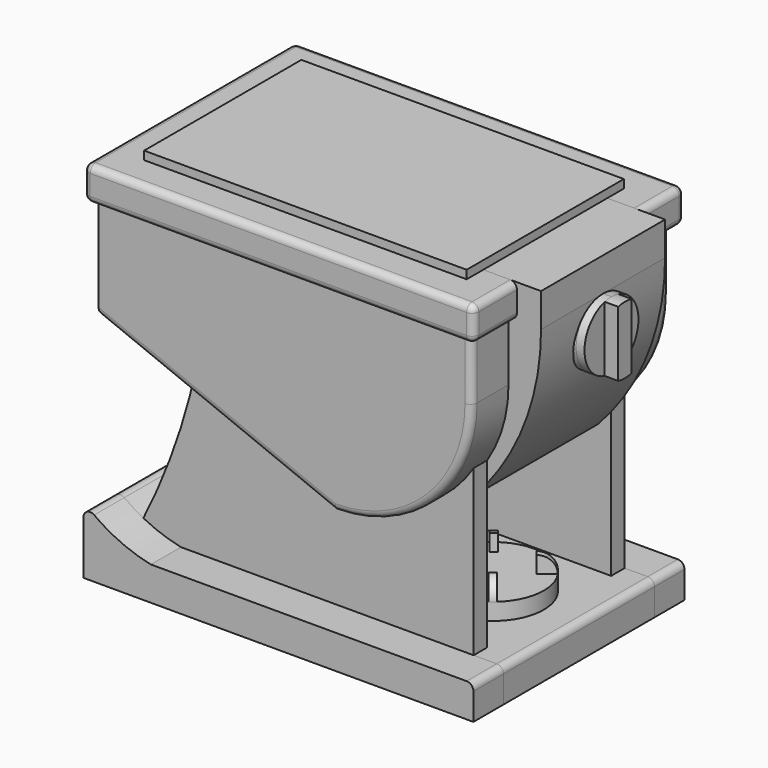
from build123d import *

# Parameters (mm, degrees)
F1_DEPTH       = 25.4
F2_W           = 140.589
F2_H           = 76.2
F3_DEPTH       = 93.091
F3_DEPTH_BACK  = 93.091
F5_DEPTH       = 99.441
F5_DEPTH_BACK  = 99.441
F4_W           = 124.46
F4_H           = 224.282
F6_DEPTH       = 71.12
F6_DEPTH_BACK  = 71.12
F7_R           = 103.37799
F9_R           = 5.08
F10_T1_DEPTH   = 203.3103950373
F10_T3_DEPTH   = 217.1807652608
F10_T5_DEPTH   = 44.70401
F10_T7_DEPTH   = 12.70001
F10_T10_ANGLE  = 90
F10_T12_ANGLE  = 90
F10_2_F1_R     = 5.08
F10_2_F2_R     = 5.08
F10_3_F1_R     = 5.08
F10_3_F2_R     = 5.08
F11_W          = 243.078
F11_H          = 148.082
F12_DEPTH      = 6.35
F13_DEPTH      = 101.6
F13_DEPTH_BACK = 25.4
F14_W          = 165.1
F14_H          = 25.4
F15_DEPTH      = 58.42
F15_DEPTH_BACK = 58.42
F17_DEPTH      = 6.35
F17_DEPTH_BACK = 25.4
F19_DEPTH      = 10.16
F21_DEPTH      = 12.7
F23_DEPTH      = 12.7
F24_T2_ANGLE   = 103.1383500352
F24_T4_ANGLE   = 103.1383500352
F24_T6_ANGLE   = 103.1383500352
F24_T8_ANGLE   = 103.1383500352


# Not quite as in the source:
# - a fillet or chamfer that OpenCascade refuses, or shapes differently, is made with other operations: its cross-section is extruded or revolved along the edge and cut away or added
# - a fillet or chamfer is up to 0.001 mm smaller than in the source, because OpenCascade refuses the exact size


with BuildPart() as f1:
    # F0 (on Top) → F1 (new body)
    with BuildSketch(Plane.XY):
        Polygon((146.939, 99.441), (0, 99.441), (-146.939, 99.441), (-146.939, 0), (-146.939, -99.441), (0, -99.441), (146.939, -99.441), (146.939, 0), align=None)
    extrude(amount=F1_DEPTH)

    # F2 (on Front) → F3 (join, two sides)
    with BuildSketch(Plane.XZ) as f3_sk:
        with Locations((-70.2945, -38.1)):
            Rectangle(F2_W, F2_H)
        Polygon((140.589, 0), (0, 0), (0, -76.2), (-140.589, -76.2), (37.211, -148.082), (140.589, -148.082), align=None)
    extrude(amount=F3_DEPTH)
    extrude(f3_sk.sketch, amount=-F3_DEPTH_BACK)

    # F7 (radius 103.378 in the source; OpenCascade refuses exactly that, so slightly less here)
    f7_edges = [f1.edges().sort_by_distance(p)[0] for p in [
        (140.589, 0, -148.082),
    ]]
    fillet(f7_edges, radius=F7_R)

    # F9
    f9_edges = [f1.edges().sort_by_distance(p)[0] for p in [
        (0, 99.441, 25.4),
        (-146.939, 0, 25.4),
        (0, -99.441, 25.4),
        (146.939, 0, 25.4),
        (0, -99.441, 0),
        (-146.939, 0, 0),
        (146.939, -99.441, 12.7),
        (146.939, 99.441, 12.7),
        (146.939, 0, 0),
        (-146.939, 99.441, 12.7),
        (-146.939, -99.441, 12.7),
        (0, 99.441, 0),
    ]]
    fillet(f9_edges, radius=F9_R)

    # F10: fillet of radius 5.08 on 7 edges, made by hand

    # F10_s2 → F10_t1 (cut)
    with BuildSketch(Plane.XZ.offset(-101.6551975186)):
        with BuildLine():
            ThreePointArc((-140.589, -72.7743209925), (-139.7208276576, -75.6145512267), (-137.4130520539, -77.4839903839))
            Line((-137.4130520539, -77.4839903839), (-140.589, -76.2))
            Line((-140.589, -76.2), (-140.589, -72.7743209925))
        make_face()
    extrude(amount=F10_T1_DEPTH, mode=Mode.SUBTRACT)

    # F10_s4 → F10_t3 (cut)
    with BuildSketch(Plane(origin=(-106.1338085529, 0, 42.9083826007), x_dir=(0, 1, 0), z_dir=(0.9271002739, 0, -0.3748133964))):
        with BuildLine():
            ThreePointArc((-93.091, -118.259681463), (-91.6031024484, -121.8517839115), (-88.011, -123.339681463))
            Line((-88.011, -123.339681463), (-93.091, -123.339681463))
            Line((-93.091, -123.339681463), (-93.091, -118.259681463))
        make_face()
        with BuildLine():
            ThreePointArc((93.091, -118.259681463), (91.6031024484, -121.8517839115), (88.011, -123.339681463))
            Line((88.011, -123.339681463), (93.091, -123.339681463))
            Line((93.091, -123.339681463), (93.091, -118.259681463))
        make_face()
    extrude(amount=F10_T3_DEPTH, mode=Mode.SUBTRACT)

    # F10_s6 → F10_t5 (cut)
    with BuildSketch(Plane.XY.offset(-44.70401)):
        with BuildLine():
            ThreePointArc((135.509, -93.091), (139.1011024484, -91.6031024484), (140.589, -88.011))
            Line((140.589, -88.011), (140.589, -93.091))
            Line((140.589, -93.091), (135.509, -93.091))
        make_face()
        with BuildLine():
            ThreePointArc((140.589, 88.011), (139.1011024484, 91.6031024484), (135.509, 93.091))
            Line((135.509, 93.091), (140.589, 93.091))
            Line((140.589, 93.091), (140.589, 88.011))
        make_face()
    extrude(amount=F10_T5_DEPTH, mode=Mode.SUBTRACT)

    # F10_s8 → F10_t7 (cut)
    with BuildSketch(Plane.YZ.offset(24.511)):
        with BuildLine():
            ThreePointArc((-93.091, -143.002), (-91.6031024484, -146.5941024484), (-88.011, -148.082))
            Line((-88.011, -148.082), (-93.091, -148.082))
            Line((-93.091, -148.082), (-93.091, -143.002))
        make_face()
        with BuildLine():
            ThreePointArc((93.091, -143.002), (91.6031024484, -146.5941024484), (88.011, -148.082))
            Line((88.011, -148.082), (93.091, -148.082))
            Line((93.091, -148.082), (93.091, -143.002))
        make_face()
    extrude(amount=F10_T7_DEPTH, mode=Mode.SUBTRACT)

    # F10_s9 → F10_t10 (revolve, cut)
    with BuildSketch(Plane.XY.offset(-44.70401)):
        with BuildLine():
            ThreePointArc((135.509, 93.091), (139.1011024484, 91.6031024484), (140.589, 88.011))
            Line((140.589, 88.011), (140.589, 93.091))
            Line((140.589, 93.091), (135.509, 93.091))
        make_face()
    revolve(axis=Axis((37.21101, 93.091, -44.70401), (0, 1, 0)), revolution_arc=F10_T10_ANGLE, mode=Mode.SUBTRACT)

    # F10_s11 → F10_t12 (revolve, cut)
    with BuildSketch(Plane.XY.offset(-44.70401)):
        with BuildLine():
            ThreePointArc((135.509, -93.091), (139.1011024484, -91.6031024484), (140.589, -88.011))
            Line((140.589, -88.011), (140.589, -93.091))
            Line((140.589, -93.091), (135.509, -93.091))
        make_face()
    revolve(axis=Axis((37.21101, -93.091, -44.70401), (0, 1, 0)), revolution_arc=F10_T12_ANGLE, mode=Mode.SUBTRACT)

    # F11 (on face) → F12 (join)
    with BuildSketch(Plane.XY.offset(25.4)):
        Rectangle(F11_W, F11_H)
    extrude(amount=F12_DEPTH)


with BuildPart() as f5:
    # F4 (on Front) → F5 (new body, two sides)
    with BuildSketch(Plane.XZ) as f5_sk:
        with BuildLine():
            Line((124.46, -224.282), (0, -224.282))
            Line((0, -224.282), (-96.139, -224.282))
            ThreePointArc((-96.139, -224.282), (-110.6394123196, -220.2008918504), (-124.46, -214.2085002298))
            ThreePointArc((-124.46, -214.2085002298), (-136.1672030432, -207.2312186368), (-146.939, -198.882))
            Line((-146.939, -198.882), (-146.939, -249.682))
            Line((-146.939, -249.682), (0, -249.682))
            Line((0, -249.682), (146.939, -249.682))
            Line((146.939, -249.682), (146.939, -224.282))
            Line((146.939, -224.282), (124.46, -224.282))
        make_face()
    extrude(amount=F5_DEPTH)
    extrude(f5_sk.sketch, amount=-F5_DEPTH_BACK)

    # F10#2: fillet of radius 5.08 on 2 edges, made by hand

    # F10_2_f1
    f10_2_f1_edges = [f5.edges().sort_by_distance(p)[0] for p in [
        (146.939, 0, -224.282),
    ]]
    fillet(f10_2_f1_edges, radius=F10_2_F1_R)

    # F10_2_f2
    f10_2_f2_edges = [f5.edges().sort_by_distance(p)[0] for p in [
        (-146.939, 0, -198.882),
    ]]
    fillet(f10_2_f2_edges, radius=F10_2_F2_R)


with BuildPart() as f6:
    # F4 (on Front) → F6 (new body, two sides)
    with BuildSketch(Plane.XZ) as f6_sk:
        with Locations((62.23, -112.141)):
            Rectangle(F4_W, F4_H)
        with BuildLine():
            Line((0, -224.282), (0, 0))
            Line((0, 0), (-73.66, 0))
            ThreePointArc((-73.66, 0), (-86.5337140534, -110.0748853857), (-124.46, -214.2085002298))
            ThreePointArc((-124.46, -214.2085002298), (-110.6394123196, -220.2008918504), (-96.139, -224.282))
            Line((-96.139, -224.282), (0, -224.282))
        make_face()
        with BuildLine():
            Line((124.46, -224.282), (0, -224.282))
            Line((0, -224.282), (-96.139, -224.282))
            ThreePointArc((-96.139, -224.282), (-110.6394123196, -220.2008918504), (-124.46, -214.2085002298))
            ThreePointArc((-124.46, -214.2085002298), (-136.1672030432, -207.2312186368), (-146.939, -198.882))
            Line((-146.939, -198.882), (-146.939, -249.682))
            Line((-146.939, -249.682), (0, -249.682))
            Line((0, -249.682), (146.939, -249.682))
            Line((146.939, -249.682), (146.939, -224.282))
            Line((146.939, -224.282), (124.46, -224.282))
        make_face()
    extrude(amount=F6_DEPTH)
    extrude(f6_sk.sketch, amount=-F6_DEPTH_BACK)

    # F10#3: fillet of radius 5.08 on 2 edges, made by hand

    # F10_3_f1
    f10_3_f1_edges = [f6.edges().sort_by_distance(p)[0] for p in [
        (146.939, 0, -224.282),
    ]]
    fillet(f10_3_f1_edges, radius=F10_3_F1_R)

    # F10_3_f2
    f10_3_f2_edges = [f6.edges().sort_by_distance(p)[0] for p in [
        (-146.939, 0, -198.882),
    ]]
    fillet(f10_3_f2_edges, radius=F10_3_F2_R)


with BuildPart() as f13_tool:
    # F8 (on face) → F13 (new body, two sides)
    with BuildSketch(Plane.YZ.offset(124.46)) as f13_sk:
        Polygon((-58.42, -49.7089512646), (-58.42, -224.282), (58.42, -224.282), (58.42, 0), (-58.42, 0), align=None)
    extrude(amount=-F13_DEPTH)
    extrude(f13_sk.sketch, amount=F13_DEPTH_BACK)


with BuildPart() as f1_1:
    add(f1.part)

    # F13: cut by f13_tool
    add(f13_tool.part, mode=Mode.SUBTRACT)


with BuildPart() as f6_1:
    add(f6.part)

    # F13: cut by f13_tool
    add(f13_tool.part, mode=Mode.SUBTRACT)


with BuildPart() as f15:
    # F14 (on Front) → F15 (new body, two sides)
    with BuildSketch(Plane.XZ) as f15_sk:
        with Locations((82.55, 12.7)):
            Rectangle(F14_W, F14_H)
        with BuildLine():
            Line((165.1, 0), (0, 0))
            Line((0, 0), (0, -127))
            Line((0, -127), (114.3, -127))
            ThreePointArc((114.3, -127), (151.9289826265, -68.3915930506), (165.1, 0))
        make_face()
    extrude(amount=F15_DEPTH)
    extrude(f15_sk.sketch, amount=-F15_DEPTH_BACK)


with BuildPart() as f17:
    # F16 (on face) → F17 (new body, two sides)
    with BuildSketch(Plane.YZ.offset(165.1)) as f17_sk:
        with BuildLine():
            ThreePointArc((25.4, -25.4), (17.9605122421, -7.4394877579), (0, 0))
            Line((0, 0), (0, -25.4))
            Line((0, -25.4), (25.4, -25.4))
        make_face()
        with BuildLine():
            Line((0, -25.4), (0, 0))
            ThreePointArc((0, 0), (-25.4, -25.4), (0, -50.8))
            Line((0, -50.8), (0, -25.4))
        make_face()
        with BuildLine():
            Line((25.4, -25.4), (0, -25.4))
            Line((0, -25.4), (0, -50.8))
            ThreePointArc((0, -50.8), (17.9605122421, -43.3605122421), (25.4, -25.4))
        make_face()
    extrude(amount=F17_DEPTH)
    extrude(f17_sk.sketch, amount=-F17_DEPTH_BACK)

    # F18 (on face) → F19 (join)
    with BuildSketch(Plane.YZ.offset(171.45)):
        with BuildLine():
            Line((-6.35, -0.8065557516), (-6.35, -49.9934442484))
            ThreePointArc((-6.35, -49.9934442484), (-3.96e-08, -50.8), (6.3499999233, -49.9934442682))
            Line((6.3499999233, -49.9934442682), (6.3499999233, -0.8065557318))
            ThreePointArc((6.3499999233, -0.8065557318), (-3.96e-08, 0), (-6.35, -0.8065557516))
        make_face()
    extrude(amount=F19_DEPTH)


with BuildPart() as f21:
    # F20 (on face) → F21 (new body)
    with BuildSketch(Plane.XY.offset(-224.282)):
        with BuildLine():
            ThreePointArc((120.4595, 0), (82.3595, 38.1), (44.2595, 0))
            Line((44.2595, 0), (120.4595, 0))
        make_face()
        with BuildLine():
            Line((120.4595, 0), (44.2595, 0))
            ThreePointArc((44.2595, 0), (82.3595, -38.1), (120.4595, 0))
        make_face()
    extrude(amount=F21_DEPTH)

    # F22 (on face) → F23 (join)
    with BuildSketch(Plane.XY.offset(-211.582)):
        with BuildLine():
            Line((96.024808986, -21.5608657135), (103.8049090505, -31.4913389785))
            ThreePointArc((103.8049090505, -31.4913389785), (105.8566221149, -29.9915863588), (107.8037872317, -28.3583893632))
            Line((107.8037872317, -28.3583893632), (100.0236871672, -18.4279160982))
            Line((100.0236871672, -18.4279160982), (96.024808986, -21.5608657135))
        make_face()
        with BuildLine():
            Line((100.7874160982, 17.6641871672), (103.9203657135, 13.665308986))
            Line((103.9203657135, 13.665308986), (113.8508389785, 21.4454090505))
            ThreePointArc((113.8508389785, 21.4454090505), (112.3510863588, 23.4971221149), (110.7178893632, 25.4442872317))
            Line((110.7178893632, 25.4442872317), (100.7874160982, 17.6641871672))
        make_face()
        with BuildLine():
            Line((54.0011106368, -25.4442872317), (63.9315839018, -17.6641871672))
            Line((63.9315839018, -17.6641871672), (60.7986342865, -13.665308986))
            Line((60.7986342865, -13.665308986), (50.8681610215, -21.4454090505))
            ThreePointArc((50.8681610215, -21.4454090505), (52.3679136412, -23.4971221149), (54.0011106368, -25.4442872317))
        make_face()
        with BuildLine():
            Line((64.6953128328, 18.4279160982), (68.694191014, 21.5608657135))
            Line((68.694191014, 21.5608657135), (60.9140909495, 31.4913389785))
            ThreePointArc((60.9140909495, 31.4913389785), (58.8623778851, 29.9915863588), (56.9152127683, 28.3583893632))
            Line((56.9152127683, 28.3583893632), (64.6953128328, 18.4279160982))
        make_face()
    extrude(amount=F23_DEPTH)

    # F24: fillet of radius 12.7 on 4 edges, made by hand

    # F24_s1 → F24_t2 (revolve, cut)
    with BuildSketch(Plane(origin=(4.4831033462, 18.684965465, 0), x_dir=(0, 0, 1), z_dir=(-0.2333095546, -0.9724025153, 0))):
        with BuildLine():
            ThreePointArc((-211.582, -118.1865849578), (-202.6017438789, -114.4668410789), (-198.882, -105.4865849578))
            Line((-198.882, -105.4865849578), (-198.882, -118.1865849578))
            Line((-198.882, -118.1865849578), (-211.582, -118.1865849578))
        make_face()
    revolve(axis=Axis((82.3595, 0, -198.882), (0, 0, 1)), revolution_arc=F24_T2_ANGLE, mode=Mode.SUBTRACT)

    # F24_s3 → F24_t4 (revolve, cut)
    with BuildSketch(Plane(origin=(77.8763966538, -18.684965465, 0), x_dir=(0, 0, 1), z_dir=(0.9724025153, -0.2333095546, 0))):
        with BuildLine():
            ThreePointArc((-211.582, -57.3152582611), (-202.6017438789, -53.5955143822), (-198.882, -44.6152582611))
            Line((-198.882, -44.6152582611), (-198.882, -57.3152582611))
            Line((-198.882, -57.3152582611), (-211.582, -57.3152582611))
        make_face()
    revolve(axis=Axis((82.3595, 0, -198.882), (0, 0, 1)), revolution_arc=F24_T4_ANGLE, mode=Mode.SUBTRACT)

    # F24_s5 → F24_t6 (revolve, cut)
    with BuildSketch(Plane(origin=(77.8763966538, -18.684965465, 0), x_dir=(0, 0, 1), z_dir=(-0.9724025153, 0.2333095546, 0))):
        with BuildLine():
            ThreePointArc((-211.582, -18.8847417389), (-202.6017438789, -15.1649978599), (-198.882, -6.1847417389))
            Line((-198.882, -6.1847417389), (-198.882, -18.8847417389))
            Line((-198.882, -18.8847417389), (-211.582, -18.8847417389))
        make_face()
    revolve(axis=Axis((82.3595, 0, -198.882), (0, 0, 1)), revolution_arc=F24_T6_ANGLE, mode=Mode.SUBTRACT)

    # F24_s7 → F24_t8 (revolve, cut)
    with BuildSketch(Plane(origin=(4.4831033462, 18.684965465, 0), x_dir=(0, 0, 1), z_dir=(0.2333095546, 0.9724025153, 0))):
        with BuildLine():
            ThreePointArc((-211.582, 41.9865849578), (-202.6017438789, 45.7063288368), (-198.882, 54.6865849578))
            Line((-198.882, 54.6865849578), (-198.882, 41.9865849578))
            Line((-198.882, 41.9865849578), (-211.582, 41.9865849578))
        make_face()
    revolve(axis=Axis((82.3595, 0, -198.882), (0, 0, 1)), revolution_arc=F24_T8_ANGLE, mode=Mode.SUBTRACT)


solid = Compound([f5.part, f1_1.part, f6_1.part, f15.part, f17.part, f21.part])
